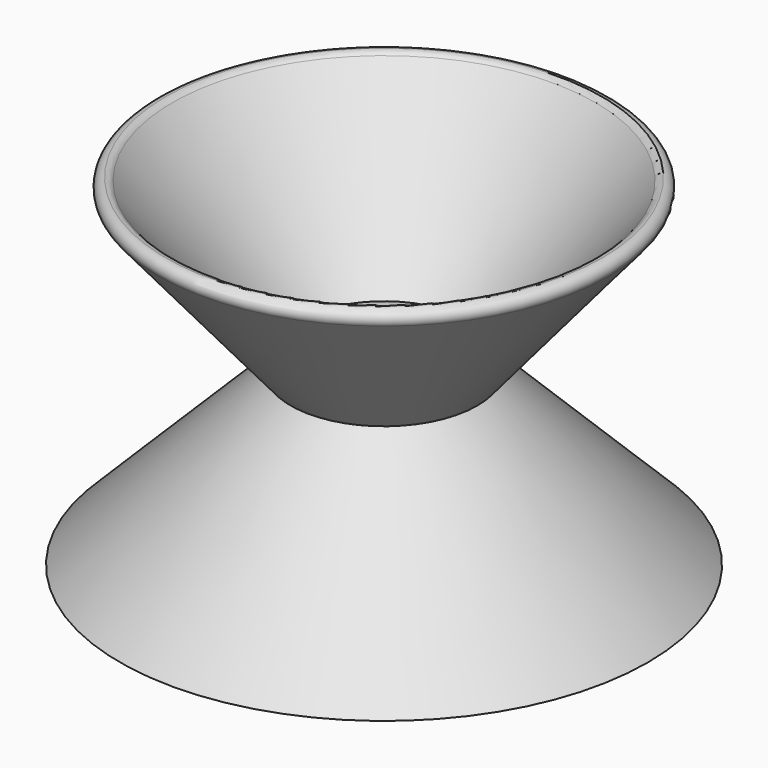
from build123d import *

# Parameters (mm, degrees)
F0_R      = 34.7636302152
F1_DEPTH  = 63.5
F1_TAPER  = -40
F2_T      = -6.35
F3_R      = 3.17499
F1_FACE_R = 34.7636302152
F4_DEPTH  = 63.5
F4_TAPER  = -45
F5_T      = -6.35


# Not quite as in the source:
# - a fillet or chamfer is up to 0.001 mm smaller than in the source, because OpenCascade refuses the exact size


with BuildPart() as f1:
    # F0 (on Top) → F1 (new body)
    with BuildSketch(Plane.XY):
        Circle(F0_R)
    extrude(amount=F1_DEPTH, taper=F1_TAPER)

    # F2
    f2_openings = [f1.faces().sort_by_distance(p)[0] for p in [
        (0, 0, 63.5),
    ]]
    offset(amount=F2_T, openings=f2_openings, kind=Kind.INTERSECTION)

    # F3 (radius 3.175 in the source; OpenCascade refuses exactly that, so slightly less here)
    f3_edges = [f1.edges().sort_by_distance(p)[0] for p in [
        (-88.046457, 0, 63.5),
        (-79.757121, 0, 63.5),
    ]]
    fillet(f3_edges, radius=F3_R)

    # F1_face (on face) → F4 (join)
    with BuildSketch(Plane(origin=(0, 0, 0), x_dir=(1, 0, 0), z_dir=(0, 0, -1))):
        Circle(F1_FACE_R)
    extrude(amount=F4_DEPTH, taper=F4_TAPER)

    # F5
    f5_openings = [f1.faces().sort_by_distance(p)[0] for p in [
        (0, 0, -63.5),
    ]]
    offset(amount=F5_T, openings=f5_openings, kind=Kind.INTERSECTION)


solid = f1.part
